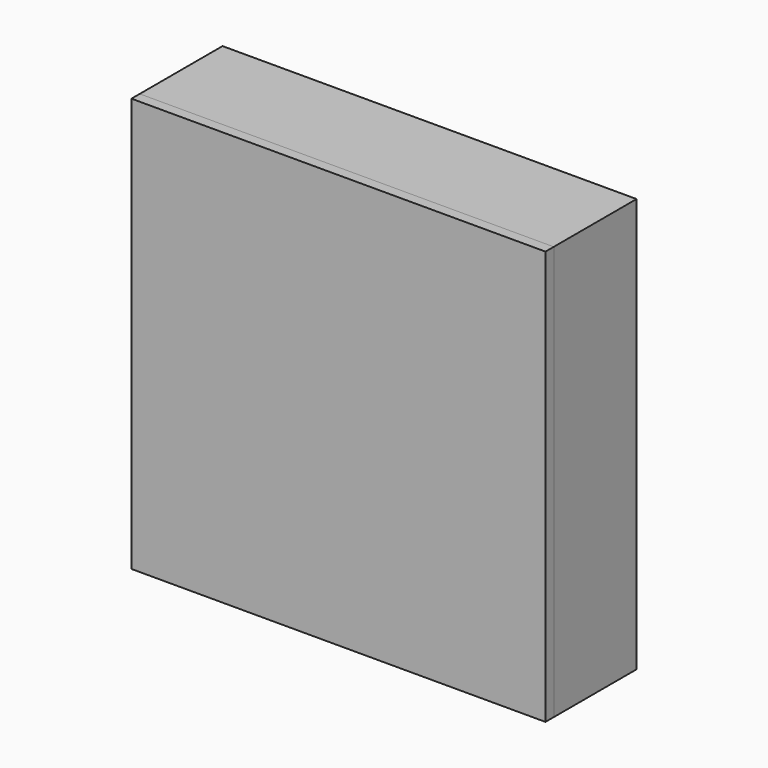
from build123d import *

# Parameters (mm, degrees)
F0_W     = 101.6
F0_H     = 101.6
F1_DEPTH = 25.4
F5_T     = -2.54
F2_W     = 96.52
F2_H     = 96.52
F2_W_2   = 93.98
F2_H_2   = 93.98
F3_DEPTH = 12.7
F6_DEPTH = 12.7
F4_W     = 101.6
F4_H     = 101.6
F4_W_2   = 96.52
F4_H_2   = 96.52
F7_DEPTH = 2.54


with BuildPart() as f1:
    # F0 (on Front) → F1 (new body)
    with BuildSketch(Plane.XZ):
        Rectangle(F0_W, F0_H)
    extrude(amount=F1_DEPTH)

    # F5
    f5_openings = [f1.faces().sort_by_distance(p)[0] for p in [
        (0, -25.4, 0),
    ]]
    offset(amount=F5_T, openings=f5_openings)

    # F2 (on face) → F3 (join)
    with BuildSketch(Plane.XZ.offset(2.54)):
        Rectangle(F2_W, F2_H)
        Rectangle(F2_W_2, F2_H_2, mode=Mode.SUBTRACT)
    extrude(amount=F3_DEPTH)


with BuildPart() as f6:
    # F6 (new): a face of the model
    f6_faces = [f1.part.faces().sort_by_distance(p)[0] for p in [
        (-48.123500107, -15.24, 0),
    ]]
    extrude(f6_faces, amount=F6_DEPTH)

    # F4 (on face) → F7 (join)
    with BuildSketch(Plane.XZ.offset(25.4)):
        Rectangle(F4_W, F4_H)
        Rectangle(F4_W_2, F4_H_2)
    extrude(amount=F7_DEPTH)


solid = Compound([f1.part, f6.part])
